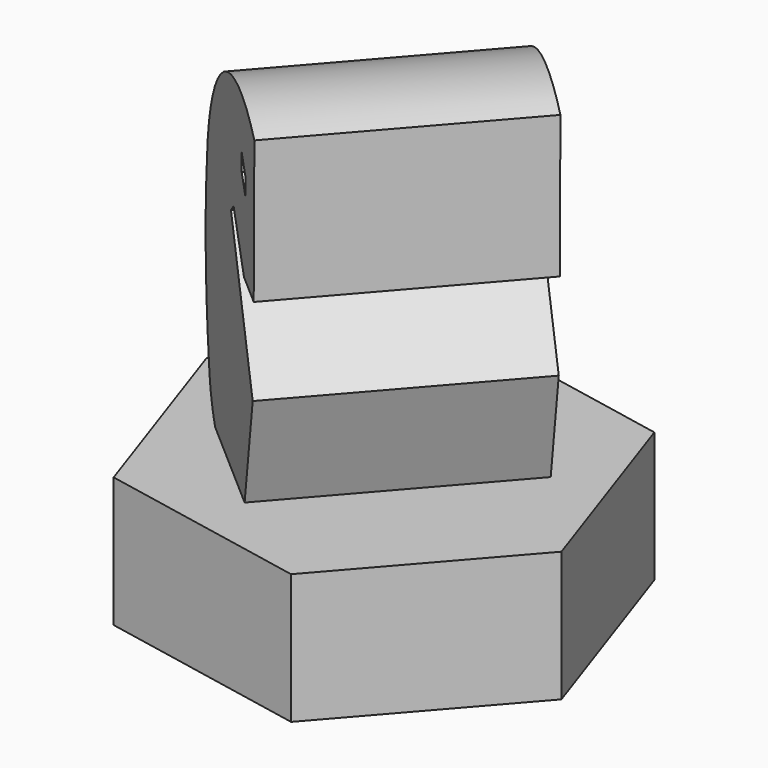
from build123d import *

# Parameters (mm, degrees)
F1_DEPTH = 17.78
F3_DEPTH = 50.8
F5_DEPTH = 76.2
F7_DEPTH = 177.8
F8_DEPTH = 177.8


# Not quite as in the source:
# - a feature names something its author has since deleted; it is built from what else it names


with BuildPart() as f1:
    # F0 (on Top) → F1 (new body)
    with BuildSketch(Plane.XY):
        Polygon((-9.4930937983, 27.7505766331), (-28.7792512331, 5.6540279267), (-19.2861574348, -22.0965487064), (9.4930937983, -27.7505766331), (28.7792512331, -5.6540279267), (19.2861574348, 22.0965487064), align=None)
    extrude(amount=F1_DEPTH)

    # F2 (on face) → F3 (join)
    with BuildSketch(Plane.XY.offset(17.78)):
        Polygon((-1.5908913392, 23.4257021287), (-23.4257021287, -1.5908913392), (1.5908913392, -23.4257021287), (23.4257021287, 1.5908913392), align=None)
    extrude(amount=F3_DEPTH)

    # F4 (on face) → F5 (cut)
    with BuildSketch(Plane(origin=(-10.9174053947, -12.508296734, 0), x_dir=(0.7533926187, -0.6575709559, 0), z_dir=(-0.6575709559, -0.7533926187, 0))):
        with BuildLine():
            Line((0, 48.7790480256), (13.0695169792, 32.4794128537))
            Line((13.0695169792, 32.4794128537), (8.2184774801, 17.78))
            Line((8.2184774801, 17.78), (16.6026271336, 17.78))
            Line((16.6026271336, 17.78), (16.6026271336, 68.58))
            Line((16.6026271336, 68.58), (-16.6026271336, 68.58))
            Line((-16.6026271336, 68.58), (-16.6026271336, 17.78))
            Line((-16.6026271336, 17.78), (-9.5075005665, 17.78))
            ThreePointArc((-9.5075005665, 17.78), (-11.8387691089, 20.1965691968), (-13.1141533635, 23.3026945488))
            ThreePointArc((-13.1141533635, 23.3026945488), (-15.1729749394, 35.6082188112), (-14.361799588, 48.0583862079))
            ThreePointArc((-14.361799588, 48.0583862079), (-4.2065001242, 63.2907896054), (14.0689240854, 64.3701831512))
            Line((14.0689240854, 64.3701831512), (13.6791784316, 44.722918421))
            Line((13.6791784316, 44.722918421), (7.8148273751, 44.722918421))
            Line((7.8148273751, 44.722918421), (1.6052529907, 50.0661861116))
            Line((1.6052529907, 50.0661861116), (0, 48.7790480256))
        make_face()
    extrude(amount=-F5_DEPTH, mode=Mode.SUBTRACT)

    # F6 (on face) → F7 (cut)
    with BuildSketch(Plane(origin=(-10.9174053947, -12.508296734, 0), x_dir=(0.7533926187, -0.6575709559, 0), z_dir=(-0.6575709559, -0.7533926187, 0))):
        Polygon((8.6703589186, 57.2541877627), (6.4581842162, 59.0407550335), (6.4581842162, 56.6472448409), (8.6703589186, 54.8606775701), align=None)
    extrude(amount=-F7_DEPTH, mode=Mode.SUBTRACT)

    # F6 (on face) → F8 (cut)
    with BuildSketch(Plane(origin=(-10.9174053947, -12.508296734, 0), x_dir=(0.7533926187, -0.6575709559, 0), z_dir=(-0.6575709559, -0.7533926187, 0))):
        Polygon((8.6703589186, 57.2541877627), (6.4581842162, 59.0407550335), (6.4581842162, 56.6472448409), (8.6703589186, 54.8606775701), align=None)
    extrude(amount=-F8_DEPTH, mode=Mode.SUBTRACT)


solid = f1.part
